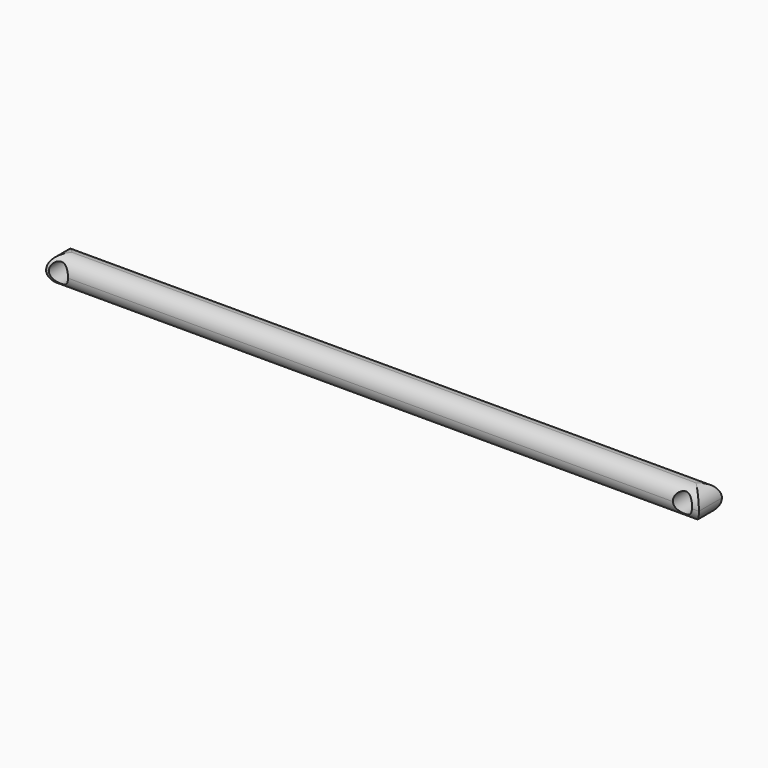
from build123d import *
from build123d import SkipClean  # not in build123d's __all__

# Parameters (mm, degrees)
F0_W        = 340
F0_H        = 15
F1_DEPTH    = 15
F2_R        = 5
F3_DEPTH    = 20
F4_T1_DEPTH = 377.5
F4_T3_DEPTH = 52.5


# Not quite as in the source:
# - a fillet or chamfer that OpenCascade refuses, or shapes differently, is made with other operations: its cross-section is extruded or revolved along the edge and cut away or added


with BuildPart() as f1:
    # F0 (on Front) → F1 (new body)
    with BuildSketch(Plane.XZ):
        with Locations((-170, 7.5)):
            Rectangle(F0_W, F0_H)
    extrude(amount=F1_DEPTH)

    # F2 (on Front) → F3 (cut)
    with BuildSketch(Plane.XZ):
        with Locations((-333.5605150089, 7.6230808641)):
            Circle(F2_R)
        with Locations((-8.5605150089, 7.8990953043)):
            Circle(F2_R)
    extrude(amount=F3_DEPTH, mode=Mode.SUBTRACT)

    # F4: fillet of radius 7.5 on 8 edges, made by hand

    # F4_s2 → F4_t1 (cut)
    with BuildSketch(Plane.YZ.offset(-358.75)):
        with BuildLine():
            ThreePointArc((-7.5, 15), (-2.1966991411, 12.8033008589), (0, 7.5))
            Line((0, 7.5), (0, 15))
            Line((0, 15), (-7.5, 15))
        make_face()
        with BuildLine():
            ThreePointArc((0, 7.5), (-2.1966991411, 2.1966991411), (-7.5, 0))
            Line((-7.5, 0), (0, 0))
            Line((0, 0), (0, 7.5))
        make_face()
        with BuildLine():
            ThreePointArc((-7.5, 15), (-12.8033008589, 12.8033008589), (-15, 7.5))
            Line((-15, 7.5), (-15, 15))
            Line((-15, 15), (-7.5, 15))
        make_face()
        with BuildLine():
            ThreePointArc((-15, 7.5), (-12.8033008589, 2.1966991411), (-7.5, 0))
            Line((-7.5, 0), (-15, 0))
            Line((-15, 0), (-15, 7.5))
        make_face()
    with SkipClean():  # cleaning this boolean's faces spoils the solid; the shape is the same uncleaned
        extrude(amount=F4_T1_DEPTH, mode=Mode.SUBTRACT)

    # F4_s4 → F4_t3 (cut)
    with BuildSketch(Plane.XZ.offset(-18.75)):
        with BuildLine():
            ThreePointArc((-7.5, 15), (-2.1966991411, 12.8033008589), (0, 7.5))
            Line((0, 7.5), (0, 15))
            Line((0, 15), (-7.5, 15))
        make_face()
        with BuildLine():
            ThreePointArc((0, 7.5), (-2.1966991411, 2.1966991411), (-7.5, 0))
            Line((-7.5, 0), (0, 0))
            Line((0, 0), (0, 7.5))
        make_face()
        with BuildLine():
            ThreePointArc((-332.5, 15), (-337.8033008589, 12.8033008589), (-340, 7.5))
            Line((-340, 7.5), (-340, 15))
            Line((-340, 15), (-332.5, 15))
        make_face()
        with BuildLine():
            ThreePointArc((-340, 7.5), (-337.8033008589, 2.1966991411), (-332.5, 0))
            Line((-332.5, 0), (-340, 0))
            Line((-340, 0), (-340, 7.5))
        make_face()
    with SkipClean():  # cleaning this boolean's faces spoils the solid; the shape is the same uncleaned
        extrude(amount=F4_T3_DEPTH, mode=Mode.SUBTRACT)


solid = f1.part
